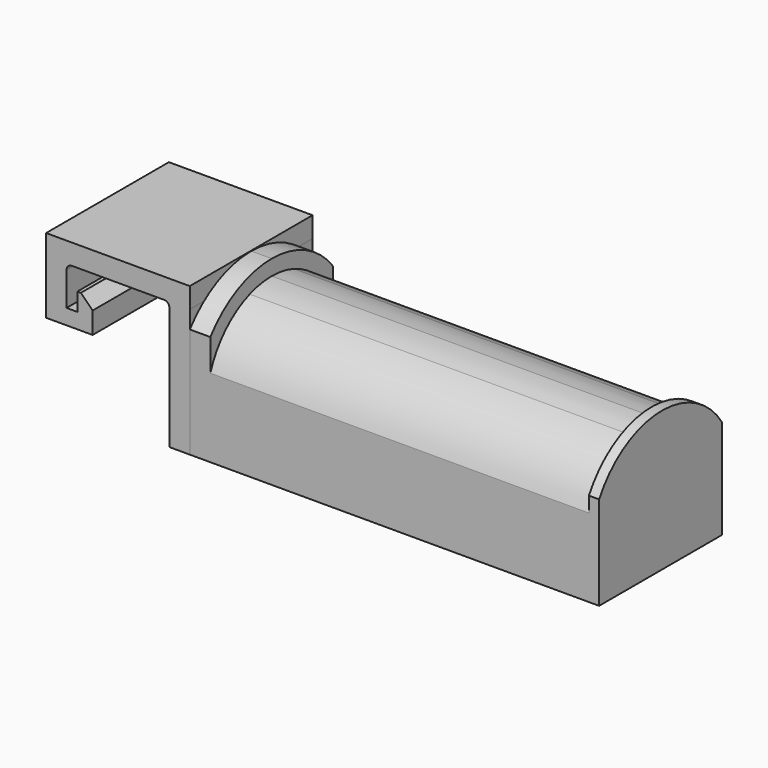
from build123d import *

# Parameters (mm, degrees)
F1_W     = 4
F1_H     = 20
F2_DEPTH = 15
F3_W     = 30
F3_H     = 15.3343126304
F4_DEPTH = 80
F5_DEPTH = 4
F7_DEPTH = 2


with BuildPart() as f2:
    # F1 (on face) → F2 (new body, symmetric)
    with BuildSketch(Plane.XZ):
        Polygon((-39.8317096115, 13.0181881455), (-42.1376643062, 15.303212098), (-42.8317096115, 15.303212098), (-42.8317096115, 11.803212098), (-42.8317096115, 8.803212098), (-39.8317096115, 8.803212098), align=None)
        Polygon((-42.8317096115, 8.803212098), (-42.8317096115, 11.803212098), (-44.9317096115, 11.803212098), (-48.9317096115, 11.803212098), (-48.9317096115, 8.803212098), align=None)
        with BuildLine():
            Line((-48.9317096115, 11.803212098), (-44.9317096115, 11.803212098))
            Line((-44.9317096115, 11.803212098), (-44.9317096115, 18.3287603771))
            ThreePointArc((-44.9317096115, 18.3287603771), (-44.6210494397, 19.0787603771), (-43.8710494397, 19.3894205489))
            Line((-43.8710494397, 19.3894205489), (-25.8317096115, 19.3894205489))
            ThreePointArc((-25.8317096115, 19.3894205489), (-25.1246028303, 19.0965273301), (-24.8317096115, 18.3894205489))
            Line((-24.8317096115, 18.3894205489), (-24.8317096115, 14.3894205489))
            Line((-24.8317096115, 14.3894205489), (-20.8317096115, 14.3894205489))
            Line((-20.8317096115, 14.3894205489), (-20.8317096115, 19.3894205489))
            Line((-20.8317096115, 19.3894205489), (-20.8479934643, 23.3894205489))
            Line((-20.8479934643, 23.3894205489), (-48.9317096115, 23.3894205489))
            Line((-48.9317096115, 23.3894205489), (-48.9317096115, 11.803212098))
        make_face()
        with Locations((-22.8317096115, 4.3894205489)):
            Rectangle(F1_W, F1_H)
    extrude(amount=F2_DEPTH, both=True)


with BuildPart() as f4:
    # F3 (on face) → F4 (new body)
    with BuildSketch(Plane.YZ.offset(-20.8317096115)):
        with BuildLine():
            ThreePointArc((-5.3753273285, 19.3894205489), (-11.2758533609, 15.6401490131), (-15, 9.7237331793))
            Line((-15, 9.7237331793), (15, 9.7237331793))
            ThreePointArc((15, 9.7237331793), (11.2758533609, 15.6401490131), (5.3753273285, 19.3894205489))
            Line((5.3753273285, 19.3894205489), (-5.3753273285, 19.3894205489))
        make_face()
        with Locations((0, 2.0565768641)):
            Rectangle(F3_W, F3_H)
        with BuildLine():
            ThreePointArc((0, 20.3248104797), (-2.7280532533, 20.0892189982), (-5.3753273285, 19.3894205489))
            Line((-5.3753273285, 19.3894205489), (5.3753273285, 19.3894205489))
            ThreePointArc((5.3753273285, 19.3894205489), (2.7280532533, 20.0892189982), (0, 20.3248104797))
        make_face()
    extrude(amount=F4_DEPTH)

    # F3 (on face) → F5 (join)
    with BuildSketch(Plane.YZ.offset(-20.8317096115)):
        with Locations((0, 2.0565768641)):
            Rectangle(F3_W, F3_H)
        with BuildLine():
            ThreePointArc((0, 20.3248104797), (-9.1839920504, 17.4070372825), (-15, 9.7237331793))
            Line((-15, 9.7237331793), (15, 9.7237331793))
            ThreePointArc((15, 9.7237331793), (9.1839920504, 17.4070372825), (0, 20.3248104797))
        make_face()
        with BuildLine():
            Line((-15, 13.3237317204), (-15, 9.7237331793))
            ThreePointArc((-15, 9.7237331793), (-9.1839920504, 17.4070372825), (0, 20.3248104797))
            ThreePointArc((0, 20.3248104797), (9.1839920504, 17.4070372825), (15, 9.7237331793))
            Line((15, 9.7237331793), (15, 13.3237317204))
            Line((15, 13.3237317204), (15, 15.9312138795))
            ThreePointArc((15, 15.9312138795), (8.3615977942, 21.376006777), (0, 23.3248104797))
            ThreePointArc((0, 23.3248104797), (-8.3615977942, 21.376006777), (-15, 15.9312138795))
            Line((-15, 15.9312138795), (-15, 13.3237317204))
        make_face()
    extrude(amount=F5_DEPTH)

    # F6 (on face) → F7 (join)
    with BuildSketch(Plane.YZ.offset(59.1682903885)):
        with BuildLine():
            Line((15, 9.7237331793), (15, 13.827643136))
            ThreePointArc((15, 13.827643136), (-0.3165064861, 21.7398244617), (-15, 12.7069399559))
            Line((-15, 12.7069399559), (-15, 9.7237331793))
            ThreePointArc((-15, 9.7237331793), (0, 20.3248104797), (15, 9.7237331793))
        make_face()
    extrude(amount=-F7_DEPTH)


solid = Compound([f2.part, f4.part])
